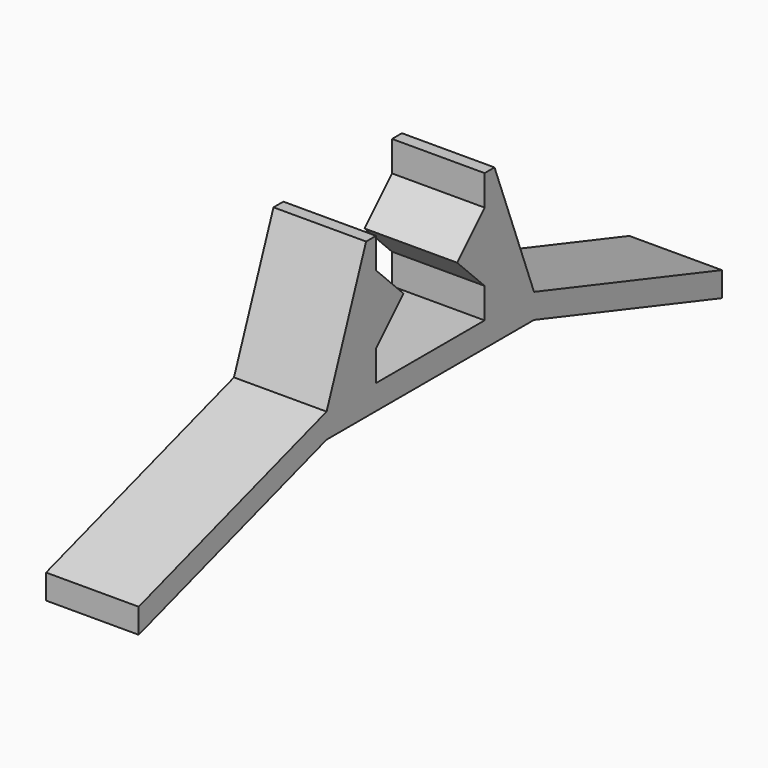
from build123d import *

# Parameters (mm, degrees)
F1_DEPTH = 15


# Not quite as in the source:
# - a feature names something its author has since deleted; it is built from what else it names


with BuildPart() as f1:
    # F0 (on Right) → F1 (new body)
    with BuildSketch(Plane.YZ):
        Polygon((5.42, 14.5), (11, 8.92), (11, 20.08), align=None)
        Polygon((-11, 20.08), (-11, 8.92), (-5.42, 14.5), align=None)
        Polygon((-21, 4), (-21, 0), (0, 0), (0, 4), (-11, 4), align=None)
        Polygon((0, 4), (0, 0), (21, 0), (21, 4), (11, 4), align=None)
        Polygon((11, 4), (21, 4), (13, 25), (11, 25), (11, 20.08), (11, 8.92), align=None)
        Polygon((-13, 25), (-21, 4), (-11, 4), (-11, 8.92), (-11, 20.08), (-11, 25), align=None)
        Polygon((21, 4), (21, 0), (59.0422606518, -12.360679775), (59.0422606518, -8.360679775), align=None)
        Polygon((-59.0422606518, -12.360679775), (-21, 0), (-21, 4), (-59.0422606518, -8.360679775), align=None)
    extrude(amount=F1_DEPTH)


solid = f1.part
